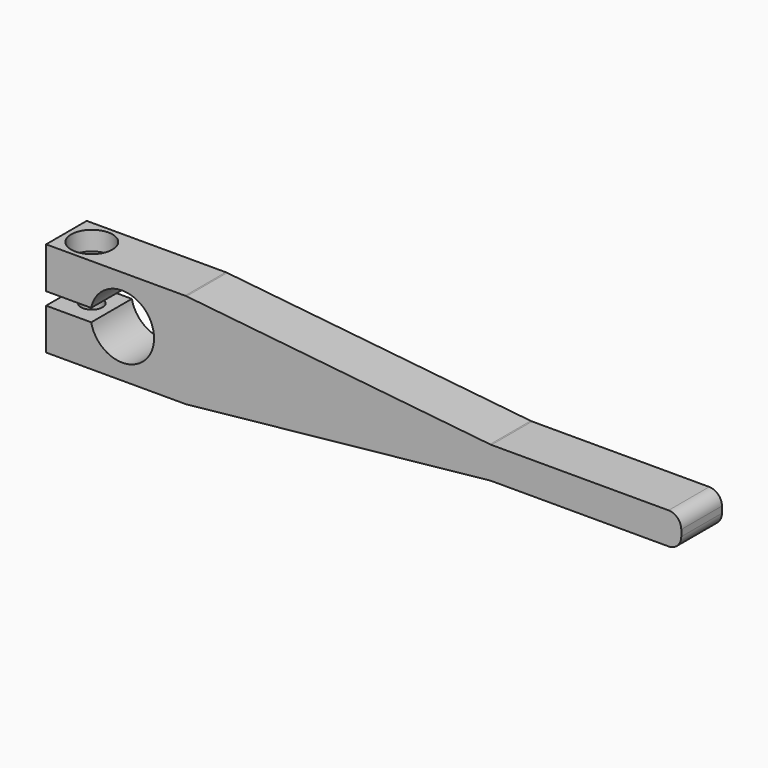
from build123d import *

# Parameters (mm, degrees)
F0_W           = 100
F0_H           = 8
F1_DEPTH       = 15
F3_DEPTH       = 8
F5_DEPTH       = 3
F7_D           = 3.4
F7_DEPTH       = 15
F7_CBORE_D     = 6.5
F7_CBORE_DEPTH = 3
F7_TIP         = 1.0214630523
F8_R           = 2


# Not quite as in the source:
# - a feature names something its author has since deleted; it is built from what else it names


with BuildPart() as f1:
    # F0 (on Top) → F1 (new body)
    with BuildSketch(Plane.XY):
        with Locations((50, 4)):
            Rectangle(F0_W, F0_H)
    extrude(amount=F1_DEPTH)

    # F2 (on face) → F3 (cut, through all)
    with BuildSketch(Plane.XZ):
        Polygon((70, 5), (22, 0), (100, 0), (100, 5), align=None)
        with BuildLine():
            Line((0, 6.5), (7.1010205144, 6.5))
            ThreePointArc((7.1010205144, 6.5), (17, 7.5), (7.1010205144, 8.5))
            Line((7.1010205144, 8.5), (0, 8.5))
            Line((0, 8.5), (0, 6.5))
        make_face()
        Polygon((100, 15), (22, 15), (70, 10), (100, 10), align=None)
    extrude(amount=-F3_DEPTH, mode=Mode.SUBTRACT)

    # F4 (on face) → F5 (cut)
    with BuildSketch(Plane(origin=(0, 0, 0), x_dir=(1, 0, 0), z_dir=(0, 0, -1))):
        Polygon((4, -7.4641016151), (7, -5.7320508076), (7, -2.2679491924), (4, -0.5358983849), (1, -2.2679491924), (1, -5.7320508076), align=None)
    extrude(amount=-F5_DEPTH, mode=Mode.SUBTRACT)

    # F7
    with Locations(Plane.XY.offset(15)):
        with Locations((4, 4)):
            CounterBoreHole(F7_D / 2, F7_CBORE_D / 2, F7_CBORE_DEPTH, depth=F7_DEPTH)
            with Locations((0, 0, -(F7_DEPTH + F7_TIP / 2))):  # 118° drill point
                Cone(0, F7_D / 2, F7_TIP, mode=Mode.SUBTRACT)

    # F8
    f8_edges = [f1.edges().sort_by_distance(p)[0] for p in [
        (100, 4, 10),
        (100, 4, 5),
        (70, 4, 5),
        (70, 4, 10),
        (22, 4, 15),
        (22, 4, 0),
    ]]
    fillet(f8_edges, radius=F8_R)


solid = f1.part
